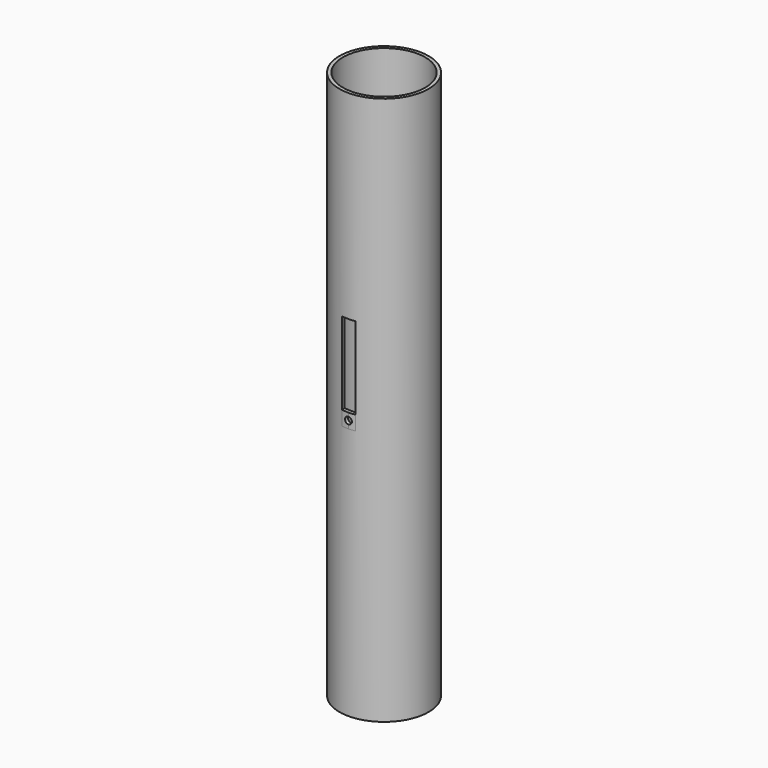
from build123d import *

# Parameters (mm, degrees)
F0_R        = 41.275
F0_R_2      = 38.1
F1_DEPTH    = 508
F3_W        = 1.5594176948
F3_H        = 13.3043527603
F4_DEPTH    = 6.35
F5_DEPTH    = 6.35
F6_R        = 3.175
F7_DEPTH    = 25.4
F8_T1_DEPTH = 52.6135854812


# Not quite as in the source:
# - a fillet or chamfer that OpenCascade refuses, or shapes differently, is made with other operations: its cross-section is extruded or revolved along the edge and cut away or added


with BuildPart() as f1:
    # F0 (on Top) → F1 (new body)
    with BuildSketch(Plane.XY):
        Circle(F0_R)
        Circle(F0_R_2, mode=Mode.SUBTRACT)
    extrude(amount=F1_DEPTH)

    # F3 (on face) → F4 (cut, symmetric)
    with BuildSketch(Plane(origin=(0, 0, 0), x_dir=(0, -1, 0), z_dir=(-1, 0, 0))):
        Polygon((63.4511685878, 247.5796341896), (63.4511685878, 323.7796341896), (25.3511685878, 323.7796341896), (25.3511685878, 247.5796341896), (39.8362353444, 247.5796341896), (41.3956530392, 247.5796341896), align=None)
        with Locations((40.6159441918, 240.9274578094)):
            Rectangle(F3_W, F3_H)
    extrude(amount=F4_DEPTH, both=True, mode=Mode.SUBTRACT)

    # F3 (on face) → F5 (join, symmetric)
    with BuildSketch(Plane(origin=(0, 0, 0), x_dir=(0, -1, 0), z_dir=(-1, 0, 0))):
        with Locations((40.6159441918, 240.9274578094)):
            Rectangle(F3_W, F3_H)
    extrude(amount=F5_DEPTH, both=True)

    # F6 (on face) → F7 (cut)
    with BuildSketch(Plane.XZ.offset(41.3956530392)):
        with Locations((0, 241.0158216953)):
            Circle(F6_R)
    extrude(amount=-F7_DEPTH, mode=Mode.SUBTRACT)

    # F8: fillet of radius 50.8 on 2 edges, made by hand

    # F8_s2 → F8_t1 (cut)
    with BuildSketch(Plane.XY.offset(214.6206650688)):
        with BuildLine():
            ThreePointArc((-6.35, -40.7836134373), (-2.4309704551, -41.2424120087), (1.5118465442, -41.3956530392))
            Line((1.5118465442, -41.3956530392), (-6.35, -41.3956530392))
            Line((-6.35, -41.3956530392), (-6.35, -40.7836134373))
        make_face()
        with BuildLine():
            ThreePointArc((6.35, -40.7836134373), (2.4309704551, -41.2424120087), (-1.5118465442, -41.3956530392))
            Line((-1.5118465442, -41.3956530392), (6.35, -41.3956530392))
            Line((6.35, -41.3956530392), (6.35, -40.7836134373))
        make_face()
    extrude(amount=F8_T1_DEPTH, mode=Mode.SUBTRACT)


solid = f1.part
